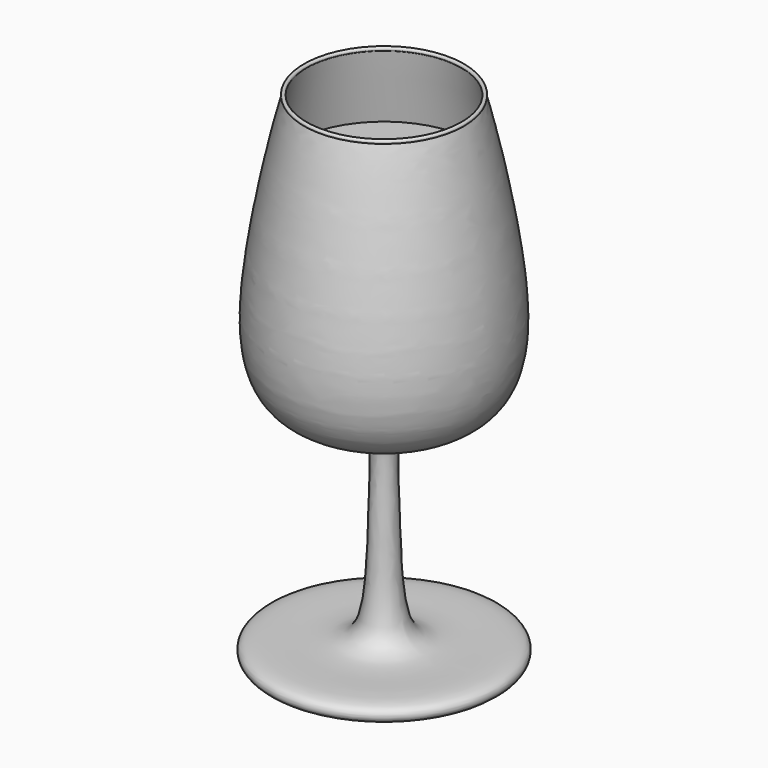
from build123d import *


with BuildPart() as f1:
    # F0 (on Front) → F1 (revolve)
    with BuildSketch(Plane.XZ):
        with BuildLine():
            Line((0, 82.9547974361), (0, 4.5005489468))
            add(Edge.make_bspline(
                [(0, 4.5005489468), (18.2505162347, 3.834930338), (34.3298208435, -1.0198899315), (45.6137322951, 0.3741983137), (45.869984667, 9.0836251174), (13.51079595, 3.614184281), (5.9426358502, 16.785848861), (5.3068801774, 43.3154798774), (3.7633712803, 78.5069717888), (7.333282914, 81.5605086481), (42.4794878758, 85.5954689569), (48.3616963183, 127.5997756572), (33.5640664678, 190.4245748965), (31.5661028946, 196.1865015243)],
                knots=[0, 0, 0, 0, 0.0803402286, 0.1174241523, 0.1430506609, 0.2129689271, 0.2590691911, 0.3294241952, 0.4054949752, 0.4302290595, 0.4992139601, 0.5871379444, 0.6856206692, 0.6856206692, 0.6856206692, 0.6856206692], degree=3))
            add(Edge.make_bspline(
                [(31.5661028946, 196.1865015243), (31.4094921747, 196.6381511386), (31.0898659276, 197.3869277296), (31.0579286187, 196.8341686094), (31.1341284742, 196.1011202354)],
                knots=[0.6856206692, 0.6856206692, 0.6856206692, 0.6856206692, 0.6933402546, 0.706037297, 0.706037297, 0.706037297, 0.706037297], degree=3))
            add(Edge.make_bspline(
                [(31.1341284742, 196.1011202354), (31.1370526235, 196.0729896976), (31.4921105294, 192.7485255774), (33.7332429133, 181.8205323436), (36.0968065343, 168.7710136175)],
                knots=[0.706037297, 0.706037297, 0.706037297, 0.706037297, 0.7065245426, 0.7624698935, 0.7624698935, 0.7624698935, 0.7624698935], degree=3))
            add(Edge.make_bspline(
                [(36.0968065343, 168.7710136175), (38.1860820867, 157.2358722727), (44.152433487, 121.2582163059), (41.2480892444, 87.8729431723), (6.9932630597, 83.791517948), (1.7452394882, 83.0149781289), (0, 82.9547974361)],
                knots=[0.7624698935, 0.7624698935, 0.7624698935, 0.7624698935, 0.811922869, 0.8965816529, 0.9659126303, 1, 1, 1, 1], degree=3))
        make_face()
        with BuildLine():
            add(Edge.make_bspline(
                [(31.5661028946, 196.1865015243), (31.4094921747, 196.6381511386), (31.0898659276, 197.3869277296), (31.0579286187, 196.8341686094), (31.1341284742, 196.1011202354)],
                knots=[0.6856206692, 0.6856206692, 0.6856206692, 0.6856206692, 0.6933402546, 0.706037297, 0.706037297, 0.706037297, 0.706037297], degree=3))
            ThreePointArc((31.5661028946, 196.1865015243), (31.0699500693, 197.5612687414), (31.1341284742, 196.1011202354))
        make_face()
    revolve(axis=Axis((0, 0, 104.0003970265), (0, 0, 1)))


with BuildPart() as f2:
    # F0 (on Front) → F2 (revolve)
    with BuildSketch(Plane.XZ):
        with BuildLine():
            Line((0, 168.7710136175), (0, 82.9547974361))
            add(Edge.make_bspline(
                [(36.0968065343, 168.7710136175), (38.1860820867, 157.2358722727), (44.152433487, 121.2582163059), (41.2480892444, 87.8729431723), (6.9932630597, 83.791517948), (1.7452394882, 83.0149781289), (0, 82.9547974361)],
                knots=[0.7624698935, 0.7624698935, 0.7624698935, 0.7624698935, 0.811922869, 0.8965816529, 0.9659126303, 1, 1, 1, 1], degree=3))
            Line((36.0968065343, 168.7710136175), (0, 168.7710136175))
        make_face()
    revolve(axis=Axis((0, 0, 104.0003970265), (0, 0, 1)))


solid = Compound([f1.part, f2.part])
